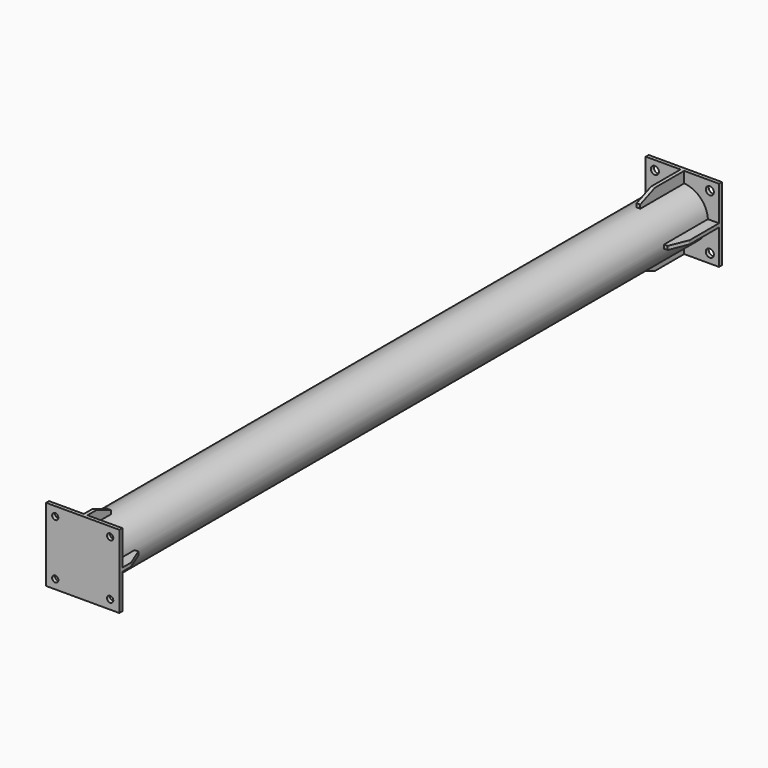
from build123d import *

# Parameters (mm, degrees)
F0_R          = 70
F0_R_2        = 65
F1_DEPTH      = 2036
F2_W          = 200
F2_H          = 200
F2_R          = 11
F3_DEPTH      = 10
F4_W          = 30.1787997812
F4_H          = 10
F4_W_2        = 10
F4_H_2        = 30.1787997812
F5_DEPTH      = 150
F6_T1_DEPTH   = 269.311363913
F6_T3_DEPTH   = 269.311363913
F6_T8_DEPTH   = 269.311363913
F6_S9_R       = 70
F6_T10_DEPTH  = 139
F8_W          = 200
F8_H          = 200
F8_R          = 8.5
F9_DEPTH      = 10
F10_W         = 10
F10_H         = 30.1787997812
F10_W_2       = 30.1787997812
F10_H_2       = 10
F11_DEPTH     = 80
F12_T1_DEPTH  = 269.311363913
F12_T3_DEPTH  = 269.311363913
F12_T8_DEPTH  = 269.311363913
F12_S9_R      = 70
F12_T10_DEPTH = 139
F12_T14_DEPTH = 269.311363913
F12_S15_R     = 70
F12_T16_DEPTH = 139


# Not quite as in the source:
# - a fillet or chamfer that OpenCascade refuses, or shapes differently, is made with other operations: its cross-section is extruded or revolved along the edge and cut away or added


with BuildPart() as f1:
    # F0 (on Front) → F1 (new body)
    with BuildSketch(Plane.XZ):
        Circle(F0_R)
        Circle(F0_R_2, mode=Mode.SUBTRACT)
    extrude(amount=F1_DEPTH)

    # F2 (on Front) → F3 (join)
    with BuildSketch(Plane.XZ):
        Rectangle(F2_W, F2_H)
        with Locations((-75, -75)):
            Circle(F2_R, mode=Mode.SUBTRACT)
        with Locations((75, -75)):
            Circle(F2_R, mode=Mode.SUBTRACT)
        with Locations((-75, 75)):
            Circle(F2_R, mode=Mode.SUBTRACT)
        with Locations((75, 75)):
            Circle(F2_R, mode=Mode.SUBTRACT)
    extrude(amount=-F3_DEPTH)

    # F4 (on Front) → F5 (join)
    with BuildSketch(Plane.XZ):
        with Locations((-84.9106001094, 0)):
            Rectangle(F4_W, F4_H)
        with Locations((0, 84.9106001094)):
            Rectangle(F4_W_2, F4_H_2)
        with Locations((84.9106001094, 0)):
            Rectangle(F4_W, F4_H)
        with Locations((0, -84.9106001094)):
            Rectangle(F4_W_2, F4_H_2)
    extrude(amount=F5_DEPTH)

    # F6: chamfer of 50 x 20 on 4 edges, made by hand

    # F6_s2 → F6_t1 (cut)
    with BuildSketch(Plane.YZ.offset(-134.6556819565)):
        Polygon((-100, 100), (-150, 80), (-150, 100), align=None)
        Polygon((-100, -100), (-150, -80), (-150, -100), align=None)
    extrude(amount=F6_T1_DEPTH, mode=Mode.SUBTRACT)

    # F6_s4 → F6_t3 (cut)
    with BuildSketch(Plane.XY.offset(-134.6556819565)):
        Polygon((100, -100), (80, -150), (100, -150), align=None)
    extrude(amount=F6_T3_DEPTH, mode=Mode.SUBTRACT)


with BuildPart() as f6_tool6:
    # F6_s7 → F6_t8 (new body)
    with BuildSketch(Plane.XY.offset(134.6556819565)):
        Polygon((-100, -130), (-50, -150), (-100, -150), align=None)
    extrude(amount=-F6_T8_DEPTH)

    # F6_s9 → F6_t10 (cut, symmetric)
    with BuildSketch(Plane.XZ.offset(140)):
        Circle(F6_S9_R)
    extrude(amount=F6_T10_DEPTH, both=True, mode=Mode.SUBTRACT)


with BuildPart() as f1_1:
    add(f1.part)

    # F6_t5: cut F6_tool6
    add(f6_tool6.part, mode=Mode.SUBTRACT)

    # F8 (on offset) → F9 (join)
    with BuildSketch(Plane.XZ.offset(2036)):
        Rectangle(F8_W, F8_H)
        with Locations((-75, -75)):
            Circle(F8_R, mode=Mode.SUBTRACT)
        with Locations((75, -75)):
            Circle(F8_R, mode=Mode.SUBTRACT)
        with Locations((-75, 75)):
            Circle(F8_R, mode=Mode.SUBTRACT)
        with Locations((75, 75)):
            Circle(F8_R, mode=Mode.SUBTRACT)
    extrude(amount=F9_DEPTH)

    # F10 (on face) → F11 (join)
    with BuildSketch(Plane(origin=(0, -2036, 0), x_dir=(-1, 0, 0), z_dir=(0, 1, 0))):
        with Locations((0, 84.9106001094)):
            Rectangle(F10_W, F10_H)
        with Locations((84.9106001094, 0)):
            Rectangle(F10_W_2, F10_H_2)
        with Locations((0, -84.9106001094)):
            Rectangle(F10_W, F10_H)
        with Locations((-84.9106001094, 0)):
            Rectangle(F10_W_2, F10_H_2)
    extrude(amount=F11_DEPTH)

    # F12: chamfer of 20 x 50 on 4 edges, made by hand

    # F12_s2 → F12_t1 (cut)
    with BuildSketch(Plane.YZ.offset(-134.6556819565)):
        Polygon((-2006, 100), (-1956, 80), (-1956, 100), align=None)
    extrude(amount=F12_T1_DEPTH, mode=Mode.SUBTRACT)

    # F12_s4 → F12_t3 (cut)
    with BuildSketch(Plane.XY.offset(-134.6556819565)):
        Polygon((100, -2006), (80, -1956), (100, -1956), align=None)
    extrude(amount=F12_T3_DEPTH, mode=Mode.SUBTRACT)


with BuildPart() as f12_tool6:
    # F12_s7 → F12_t8 (new body)
    with BuildSketch(Plane.XY.offset(-134.6556819565)):
        Polygon((-100, -1976), (-50, -1956), (-100, -1956), align=None)
    extrude(amount=F12_T8_DEPTH)

    # F12_s9 → F12_t10 (cut, symmetric)
    with BuildSketch(Plane.XZ.offset(1966)):
        Circle(F12_S9_R)
    extrude(amount=F12_T10_DEPTH, both=True, mode=Mode.SUBTRACT)


with BuildPart() as f1_2:
    add(f1_1.part)

    # F12_t5: cut F12_tool6
    add(f12_tool6.part, mode=Mode.SUBTRACT)


with BuildPart() as f12_tool12:
    # F12_s13 → F12_t14 (new body)
    with BuildSketch(Plane.YZ.offset(134.6556819565)):
        Polygon((-1976, -100), (-1956, -50), (-1956, -100), align=None)
    extrude(amount=-F12_T14_DEPTH)

    # F12_s15 → F12_t16 (cut, symmetric)
    with BuildSketch(Plane.XZ.offset(1966)):
        Circle(F12_S15_R)
    extrude(amount=F12_T16_DEPTH, both=True, mode=Mode.SUBTRACT)


with BuildPart() as f1_3:
    add(f1_2.part)

    # F12_t11: cut F12_tool12
    add(f12_tool12.part, mode=Mode.SUBTRACT)


solid = f1_3.part
